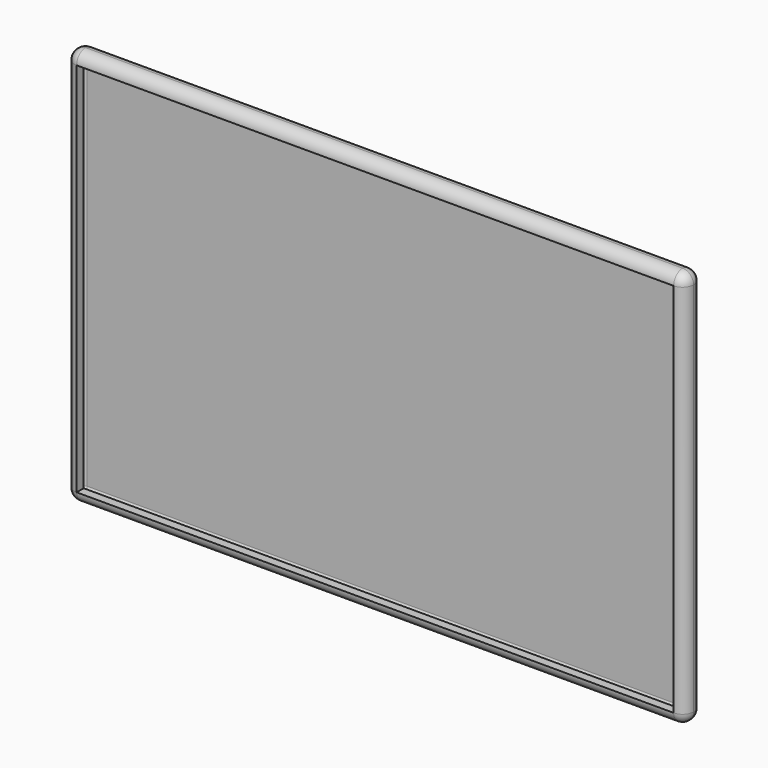
from build123d import *

# Parameters (mm, degrees)
F0_W     = 177.8
F0_H     = 114.3
F1_DEPTH = 6.35
F2_R     = 3.17499
F3_T     = -2.54


# Not quite as in the source:
# - a fillet or chamfer is up to 0.001 mm smaller than in the source, because OpenCascade refuses the exact size
# - a shell that OpenCascade refuses in one call is made with other operations: the cavity is built on its own and cut out


with BuildPart() as f1:
    # F0 (on Front) → F1 (new body)
    with BuildSketch(Plane.XZ):
        with Locations((45.9769070864, 28.9183518412)):
            Rectangle(F0_W, F0_H)
    extrude(amount=F1_DEPTH)

    # F2 (radius 3.175 in the source; OpenCascade refuses exactly that, so slightly less here)
    f2_edges = [f1.edges().sort_by_distance(p)[0] for p in [
        (45.976907, 0, 86.068352),
        (134.876907, -3.175, 86.068352),
        (45.976907, -6.35, 86.068352),
        (-42.923093, -3.175, 86.068352),
        (-42.923093, -6.35, 28.918352),
        (134.876907, -6.35, 28.918352),
        (134.876907, 0, 28.918352),
        (45.976907, -6.35, -28.231648),
        (45.976907, 0, -28.231648),
        (-42.923093, 0, 28.918352),
        (134.876907, -3.175, -28.231648),
        (-42.923093, -3.175, -28.231648),
    ]]
    fillet(f2_edges, radius=F2_R)

    # F3: a shell. OpenCascade refuses it in one call, so the cavity is built on its own and cut out:
    # the body offset inwards by the wall thickness, plus a prism from it out through each open face.
    f3_core = offset(f1.part, amount=F3_T, mode=Mode.PRIVATE)
    f3_exits = [f3_core.faces().sort_by_distance(p)[0] for p in [
        (45.976907, -3.81, 28.918352),
    ]]
    add(f3_core, mode=Mode.SUBTRACT)
    extrude(f3_exits, amount=-F3_T, mode=Mode.SUBTRACT)


solid = f1.part
